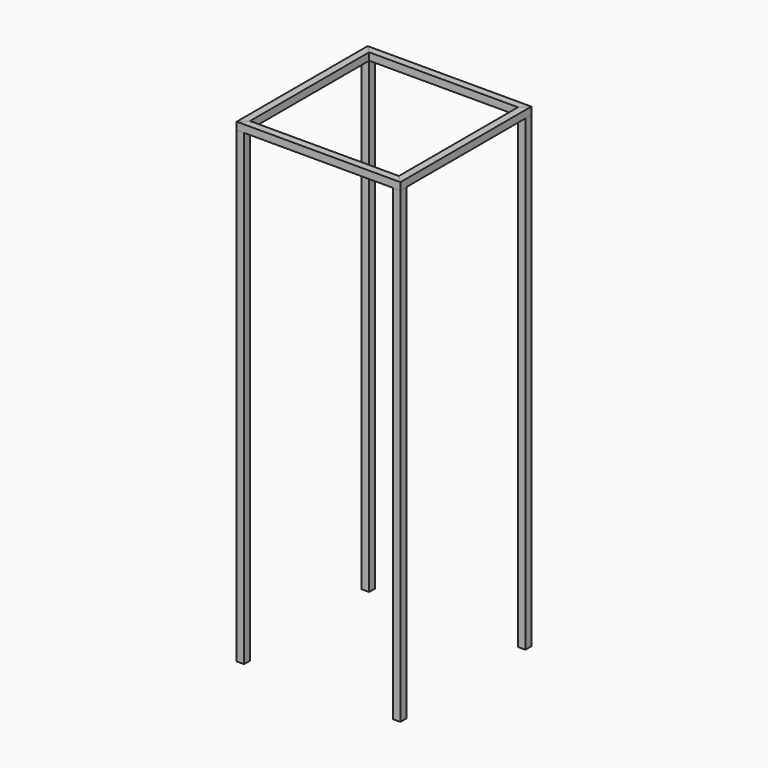
from build123d import *

# Parameters (mm, degrees)
F1_DEPTH = 3.175
F2_DEPTH = 3.175
F5_SIZE  = 3.17499
F6_ANGLE = 90
F7_ANGLE = 180


# Not quite as in the source:
# - a fillet or chamfer is up to 0.001 mm smaller than in the source, because OpenCascade refuses the exact size


with BuildPart() as f1:
    # F0 (on Front) → F1 (new body)
    with BuildSketch(Plane.XZ):
        Polygon((3.175, 200), (0, 200), (0, 0), (3.175, 0), (3.175, 91.6580334306), (3.175, 100), (3.175, 103.175), (3.175, 144.3984588309), (3.175, 148.181190443), (3.175, 151.356190443), (3.175, 183.6910381727), (3.175, 187.2522424124), (3.175, 190.4272424124), (3.175, 196.8090808041), align=None)
    extrude(amount=F1_DEPTH)


with BuildPart() as f2:
    # F0 (on Front) → F2 (new body)
    with BuildSketch(Plane.XZ):
        Polygon((0, 203.175), (0, 200), (3.175, 200), (66.825, 200), (70, 200), (70, 203.175), align=None)
    extrude(amount=F2_DEPTH)

    # F5 (size 3.175 in the source; OpenCascade refuses exactly that, so slightly less here)
    f5_edges = [f2.edges().sort_by_distance(p)[0] for p in [
        (0, -3.175, 201.5875),
        (70, -3.175, 201.5875),
    ]]
    chamfer(f5_edges, length=F5_SIZE)


with BuildPart() as f6_1:
    # F6: copy of F1
    add(f1.part.rotate(Axis((35, -35, 100), (0, 0, -1)), F6_ANGLE))


with BuildPart() as f6_2:
    # F6: copy of F2
    add(f2.part.rotate(Axis((35, -35, 100), (0, 0, -1)), F6_ANGLE))


with BuildPart() as f7_1:
    # F7: copy of F1
    add(f1.part.rotate(Axis((35, -35, 100), (0, 0, -1)), F7_ANGLE))


with BuildPart() as f7_2:
    # F7: copy of F2
    add(f2.part.rotate(Axis((35, -35, 100), (0, 0, -1)), F7_ANGLE))


with BuildPart() as f7_3:
    # F7: copy of F6_1
    add(f6_1.part.rotate(Axis((35, -35, 100), (0, 0, -1)), F7_ANGLE))


with BuildPart() as f7_4:
    # F7: copy of F6_2
    add(f6_2.part.rotate(Axis((35, -35, 100), (0, 0, -1)), F7_ANGLE))


solid = Compound([f1.part, f2.part, f6_1.part, f6_2.part, f7_1.part, f7_2.part, f7_3.part, f7_4.part])
